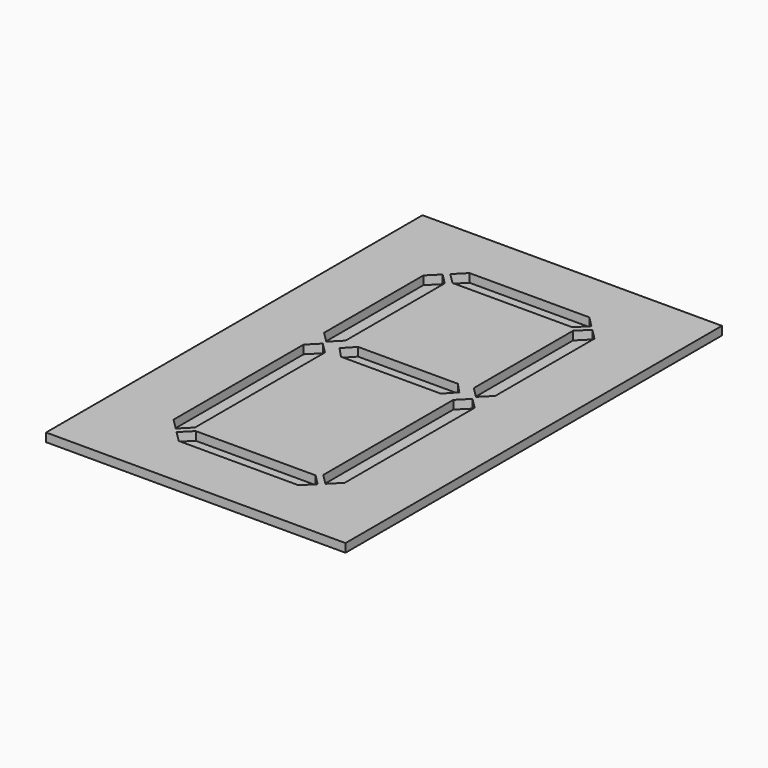
from build123d import *

# Parameters (mm, degrees)
F0_W     = 70
F0_H     = 110
F1_DEPTH = 2
F3_DEPTH = 2
F5_DEPTH = 1
F7_DEPTH = 1


# Not quite as in the source:
# - a feature names something its author has since deleted; it is built from what else it names


with BuildPart() as f1:
    # F0 (on Top) → F1 (new body)
    with BuildSketch(Plane.XY):
        with Locations((35, 55)):
            Rectangle(F0_W, F0_H)
        Polygon((20, 18.5), (17.5, 16), (15, 18.5), (15, 56.5), (17.5, 59), (20, 56.5), align=None, mode=Mode.SUBTRACT)
        Polygon((18.5, 15), (21, 17.5), (49, 17.5), (51.5, 15), (49, 12.5), (21, 12.5), align=None, mode=Mode.SUBTRACT)
        Polygon((50, 18.5), (50, 56.5), (52.5, 59), (55, 56.5), (55, 18.5), (52.5, 16), align=None, mode=Mode.SUBTRACT)
        Polygon((15, 91.5), (17.5, 94), (20, 91.5), (20, 62.5), (17.5, 60), (15, 62.5), align=None, mode=Mode.SUBTRACT)
        Polygon((23.3336448214, 57), (21, 59.5), (23.3336448214, 62), (46.6663551786, 62), (49, 59.5), (46.6663551786, 57), align=None, mode=Mode.SUBTRACT)
        Polygon((50, 91.5), (52.5, 94), (55, 91.5), (55, 62.5), (52.5, 60), (50, 62.5), align=None, mode=Mode.SUBTRACT)
        Polygon((21, 92.5), (18.5, 95), (21, 97.5), (49, 97.5), (51.5, 95), (49, 92.5), align=None, mode=Mode.SUBTRACT)
    extrude(amount=F1_DEPTH)

    # F2 (on face) → F3 (join)
    with BuildSketch(Plane(origin=(0, 0, 0), x_dir=(1, 0, 0), z_dir=(0, 0, -1))):
        Polygon((51.5, -15), (49, -17.5), (21, -17.5), (18.5, -15), (18.5, -7.5), (10, -16), (17.5, -16), (20, -18.5), (20, -56.5), (17.5, -59), (10, -59), (10, -60), (17.5, -60), (20, -62.5), (20, -91.5), (17.5, -94), (10, -94), (18.5, -102.5), (18.5, -95), (21, -92.5), (49, -92.5), (51.5, -95), (51.5, -102.5), (60, -94), (52.5, -94), (50, -91.5), (50, -62.5), (52.5, -60), (60, -60), (60, -59), (52.5, -59), (50, -56.5), (50, -18.5), (52.5, -16), (60, -16), (51.5, -7.5), align=None)
        Polygon((49, -61.0261154606), (49, -91.5), (21, -91.5), (21, -60.9654872063), (22.8991320981, -63), (47.1008679019, -63), (48.9434060753, -61.0261154606), align=None, mode=Mode.SUBTRACT)
        Polygon((21, -18.5), (49, -18.5), (49, -51.9142135624), (49, -59.5), (46.6663551786, -62), (23.3336448214, -62), (21, -59.5), (21, -51.9142135624), align=None, mode=Mode.SUBTRACT)
    extrude(amount=F3_DEPTH)

    # F4 (on face) → F5 (join)
    with BuildSketch(Plane(origin=(0, 0, -2), x_dir=(1, 0, 0), z_dir=(0, 0, -1))):
        Polygon((23.9248658717, -102.5), (23.9248658717, -97.5), (47.1921387315, -97.5), (47.1921387315, -102.5), (51.5, -102.5), (60, -94), (60, -83.6655944586), (55, -83.6655944586), (55, -65.0172777596), (60, -65.0172777596), (60, -49.3863895535), (55, -49.3863895535), (55, -21.2481319904), (60, -21.2481319904), (60, -16), (51.5, -7.5), (46.5375445783, -7.5), (46.5375445783, -12.5), (25.0055992454, -12.5), (25.0055992454, -7.5), (18.5, -7.5), (10, -16), (10, -21.093017593), (15, -21.093017593), (15, -50.3691881895), (10, -50.3691881895), (10, -65.0000932597), (15, -65.0000932597), (15, -89.8551392555), (10, -89.8551392555), (10, -94), (18.5, -102.5), align=None)
        Polygon((49, -91.5), (44.0906696022, -91.5), (21, -91.5), (21, -68.9583107835), (21, -60.9654872063), (23.1079336207, -63), (47.1008679019, -63), (49, -61.0261154606), align=None, mode=Mode.SUBTRACT)
        Polygon((21, -49.632139504), (21, -18.5), (49, -18.5), (49, -49.632139504), (43.7561757863, -49.632139504), (43.7561757863, -57), (26.6159512103, -57), (26.6159512103, -49.632139504), align=None, mode=Mode.SUBTRACT)
    extrude(amount=F5_DEPTH)


with BuildPart() as f7:
    # F6 (on face) → F7 (new body)
    with BuildSketch(Plane(origin=(0, 0, 0), x_dir=(1, 0, 0), z_dir=(0, 0, -1))):
        Polygon((49, -92.5), (21, -92.5), (18.5, -95), (18.5, -101), (51.5, -101), (51.5, -95), align=None)
    extrude(amount=F7_DEPTH)


with BuildPart() as f7b:
    # F6 (on face) → F7, piece 2 (new body)
    with BuildSketch(Plane(origin=(0, 0, 0), x_dir=(1, 0, 0), z_dir=(0, 0, -1))):
        Polygon((11.5, -94), (17.5, -94), (20, -91.5), (20, -62.5), (17.5, -60), (11.5, -60), align=None)
    extrude(amount=F7_DEPTH)


with BuildPart() as f7c:
    # F6 (on face) → F7, piece 3 (new body)
    with BuildSketch(Plane(origin=(0, 0, 0), x_dir=(1, 0, 0), z_dir=(0, 0, -1))):
        Polygon((50, -91.5), (52.5, -94), (58.5, -94), (58.5, -60), (52.5, -60), (50, -62.5), align=None)
    extrude(amount=F7_DEPTH)


with BuildPart() as f7d:
    # F6 (on face) → F7, piece 4 (new body)
    with BuildSketch(Plane(origin=(0, 0, 0), x_dir=(1, 0, 0), z_dir=(0, 0, -1))):
        Polygon((21, -53.5), (21, -59.5), (23.3336448214, -62), (46.6663551786, -62), (49, -59.5), (49, -53.5), align=None)
    extrude(amount=F7_DEPTH)


with BuildPart() as f7e:
    # F6 (on face) → F7, piece 5 (new body)
    with BuildSketch(Plane(origin=(0, 0, 0), x_dir=(1, 0, 0), z_dir=(0, 0, -1))):
        Polygon((17.5, -59), (20, -56.5), (20, -18.5), (17.5, -16), (11.5, -16), (11.5, -59), align=None)
    extrude(amount=F7_DEPTH)


with BuildPart() as f7f:
    # F6 (on face) → F7, piece 6 (new body)
    with BuildSketch(Plane(origin=(0, 0, 0), x_dir=(1, 0, 0), z_dir=(0, 0, -1))):
        Polygon((50, -18.5), (50, -56.5), (52.5, -59), (58.5, -59), (58.5, -16), (52.5, -16), align=None)
    extrude(amount=F7_DEPTH)


with BuildPart() as f7g:
    # F6 (on face) → F7, piece 7 (new body)
    with BuildSketch(Plane(origin=(0, 0, 0), x_dir=(1, 0, 0), z_dir=(0, 0, -1))):
        Polygon((18.5, -9), (18.5, -15), (21, -17.5), (49, -17.5), (51.5, -15), (51.5, -9), align=None)
    extrude(amount=F7_DEPTH)


solid = Compound([f1.part, f7.part, f7b.part, f7c.part, f7d.part, f7e.part, f7f.part, f7g.part])
